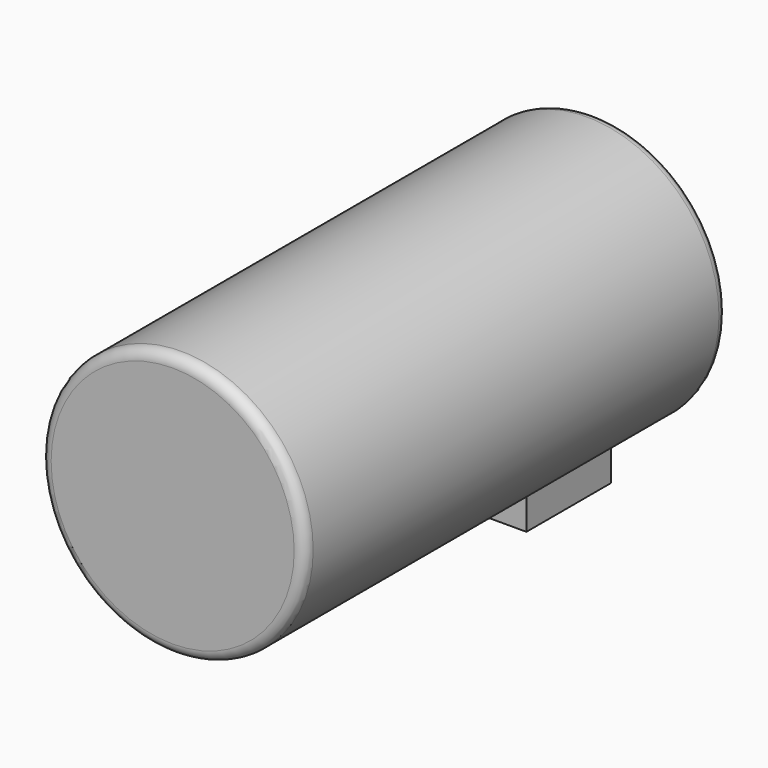
from build123d import *

# Parameters (mm, degrees)
F0_R     = 63.5
F1_DEPTH = 254
F4_R     = 5.08
F5_W     = 50.8
F5_H     = 50.8
F6_DEPTH = 76.2


# Not quite as in the source:
# - the program builds the solid bodies; features that only make, move or delete a surface that nothing else refers to are left out


with BuildPart() as f1:
    # F0 (on Front) → F1 (new body)
    with BuildSketch(Plane.XZ):
        Circle(F0_R)
    extrude(amount=F1_DEPTH)

    # F4
    f4_edges = [f1.edges().sort_by_distance(p)[0] for p in [
        (-63.5, -254, 0),
        (-63.5, 0, 0),
    ]]
    fillet(f4_edges, radius=F4_R)

    # F5 (on Top) → F6 (join)
    with BuildSketch(Plane.XY):
        with Locations((0, -47.7578863502)):
            Rectangle(F5_W, F5_H)
    extrude(amount=-F6_DEPTH)


solid = f1.part
